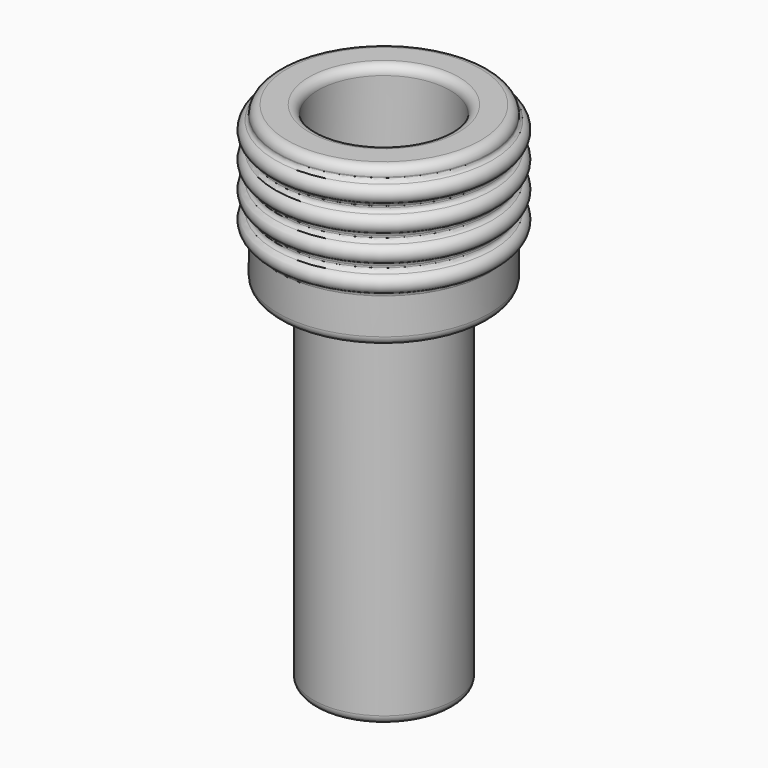
from build123d import *

# Parameters (mm, degrees)
F0_R          = 6
F0_R_2        = 2.05
F1_DEPTH      = 4
F2_R          = 6
F2_R_2        = 3.75
F3_DEPTH      = 5
F4_R          = 0.5
F5_R          = 4
F5_R_2        = 2.05
F6_DEPTH      = 20
F7_R          = 0.5
F10_T3_ANGLE  = 180
F10_T6_ANGLE  = 180
F10_T9_ANGLE  = 180
F10_T12_ANGLE = 180
F10_T15_ANGLE = 180
F10_T18_ANGLE = 180
F10_T21_ANGLE = 180
F10_T24_ANGLE = 180
F10_T27_ANGLE = 180
F10_T30_ANGLE = 180
F10_T33_ANGLE = 180
F10_T36_ANGLE = 180
F10_T39_ANGLE = 180
F10_T42_ANGLE = 180
F10_T45_ANGLE = 180
F10_T48_ANGLE = 180


# Not quite as in the source:
# - a fillet or chamfer that OpenCascade refuses, or shapes differently, is made with other operations: its cross-section is extruded or revolved along the edge and cut away or added


with BuildPart() as f1:
    # F0 (on Top) → F1 (new body)
    with BuildSketch(Plane.XY):
        Circle(F0_R)
        Circle(F0_R_2, mode=Mode.SUBTRACT)
    extrude(amount=F1_DEPTH)

    # F2 (on face) → F3 (join)
    with BuildSketch(Plane.XY.offset(4)):
        Circle(F2_R)
        Circle(F2_R_2, mode=Mode.SUBTRACT)
    extrude(amount=F3_DEPTH)

    # F4
    f4_edges = [f1.edges().sort_by_distance(p)[0] for p in [
        (-3.75, 0, 4),
        (-2.05, 0, 4),
        (-6, 0, 9),
        (-3.75, 0, 9),
    ]]
    fillet(f4_edges, radius=F4_R)

    # F5 (on face) → F6 (join)
    with BuildSketch(Plane(origin=(0, 0, 0), x_dir=(1, 0, 0), z_dir=(0, 0, -1))):
        Circle(F5_R)
        Circle(F5_R_2, mode=Mode.SUBTRACT)
    extrude(amount=F6_DEPTH)

    # F7
    f7_edges = [f1.edges().sort_by_distance(p)[0] for p in [
        (-6, 0, 0),
        (-4, 0, 0),
        (-4, 0, -20),
        (-2.05, 0, -20),
    ]]
    fillet(f7_edges, radius=F7_R)

    # F8 (on Front) → F9 (revolve)
    with BuildSketch(Plane.XZ):
        with BuildLine():
            ThreePointArc((-6, 3.75), (-6.5, 3.25), (-6, 2.75))
            Line((-6, 2.75), (-6, 3.75))
        make_face()
        with BuildLine():
            ThreePointArc((-6, 8.25), (-6.5, 7.75), (-6, 7.25))
            Line((-6, 7.25), (-6, 8.25))
        make_face()
        with BuildLine():
            Line((-6, 8.25), (-6, 7.25))
            ThreePointArc((-6, 7.25), (-5.6464466094, 7.3964466094), (-5.5, 7.75))
            ThreePointArc((-5.5, 7.75), (-5.6464466094, 8.1035533906), (-6, 8.25))
        make_face()
        with BuildLine():
            ThreePointArc((-6, 6.75), (-6.5, 6.25), (-6, 5.75))
            Line((-6, 5.75), (-6, 6.75))
        make_face()
        with BuildLine():
            Line((-6, 6.75), (-6, 5.75))
            ThreePointArc((-6, 5.75), (-5.6464466094, 5.8964466094), (-5.5, 6.25))
            ThreePointArc((-5.5, 6.25), (-5.6464466094, 6.6035533906), (-6, 6.75))
        make_face()
        with BuildLine():
            ThreePointArc((-6, 5.25), (-6.5, 4.75), (-6, 4.25))
            Line((-6, 4.25), (-6, 5.25))
        make_face()
        with BuildLine():
            Line((-6, 5.25), (-6, 4.25))
            ThreePointArc((-6, 4.25), (-5.6464466094, 4.3964466094), (-5.5, 4.75))
            ThreePointArc((-5.5, 4.75), (-5.6464466094, 5.1035533906), (-6, 5.25))
        make_face()
        with BuildLine():
            Line((-6, 3.75), (-6, 2.75))
            ThreePointArc((-6, 2.75), (-5.6464466094, 2.8964466094), (-5.5, 3.25))
            ThreePointArc((-5.5, 3.25), (-5.6464466094, 3.6035533906), (-6, 3.75))
        make_face()
    revolve(axis=Axis((0, 0, 0), (0, 0, -1)))

    # F10: fillet of radius 0.25 on 23 edges, made by hand


with BuildPart() as f10_tool1:
    # F10_s2 → F10_t3 (revolve)
    with BuildSketch(Plane.XZ):
        with BuildLine():
            ThreePointArc((-6.1666666667, 6.7214045208), (-6.0458758548, 6.8127692139), (-6, 6.9571067812))
            Line((-6, 6.9571067812), (-6, 6.75))
            ThreePointArc((-6, 6.75), (-6.0845509894, 6.7427992798), (-6.1666666667, 6.7214045208))
        make_face()
    revolve(axis=Axis((0, 0, 6.75), (0, 0, -1)), revolution_arc=F10_T3_ANGLE)


with BuildPart() as f10_tool4:
    # F10_s5 → F10_t6 (revolve)
    with BuildSketch(Plane.XZ):
        with BuildLine():
            ThreePointArc((6.1666666667, 6.7214045208), (6.0458758548, 6.8127692139), (6, 6.9571067812))
            Line((6, 6.9571067812), (6, 6.75))
            ThreePointArc((6, 6.75), (6.0845509894, 6.7427992798), (6.1666666667, 6.7214045208))
        make_face()
    revolve(axis=Axis((0, 0, 6.75), (0, 0, -1)), revolution_arc=F10_T6_ANGLE)


with BuildPart() as f10_tool7:
    # F10_s8 → F10_t9 (revolve)
    with BuildSketch(Plane.XZ):
        with BuildLine():
            ThreePointArc((6, 7.0428932188), (6.0458758548, 7.1872307861), (6.1666666667, 7.2785954792))
            ThreePointArc((6.1666666667, 7.2785954792), (6.0845509894, 7.2572007202), (6, 7.25))
            Line((6, 7.25), (6, 7.0428932188))
        make_face()
    revolve(axis=Axis((0, 0, 7.25), (0, 0, -1)), revolution_arc=F10_T9_ANGLE)


with BuildPart() as f10_tool10:
    # F10_s11 → F10_t12 (revolve)
    with BuildSketch(Plane.XZ):
        with BuildLine():
            ThreePointArc((-6, 7.0428932188), (-6.0458758548, 7.1872307861), (-6.1666666667, 7.2785954792))
            ThreePointArc((-6.1666666667, 7.2785954792), (-6.0845509894, 7.2572007202), (-6, 7.25))
            Line((-6, 7.25), (-6, 7.0428932188))
        make_face()
    revolve(axis=Axis((0, 0, 7.25), (0, 0, -1)), revolution_arc=F10_T12_ANGLE)


with BuildPart() as f10_tool13:
    # F10_s14 → F10_t15 (revolve)
    with BuildSketch(Plane.XZ):
        with BuildLine():
            ThreePointArc((-6.1666666667, 5.2214045208), (-6.0458758548, 5.3127692139), (-6, 5.4571067812))
            Line((-6, 5.4571067812), (-6, 5.25))
            ThreePointArc((-6, 5.25), (-6.0845509894, 5.2427992798), (-6.1666666667, 5.2214045208))
        make_face()
    revolve(axis=Axis((0, 0, 5.25), (0, 0, -1)), revolution_arc=F10_T15_ANGLE)


with BuildPart() as f10_tool16:
    # F10_s17 → F10_t18 (revolve)
    with BuildSketch(Plane.XZ):
        with BuildLine():
            ThreePointArc((6.1666666667, 5.2214045208), (6.0458758548, 5.3127692139), (6, 5.4571067812))
            Line((6, 5.4571067812), (6, 5.25))
            ThreePointArc((6, 5.25), (6.0845509894, 5.2427992798), (6.1666666667, 5.2214045208))
        make_face()
    revolve(axis=Axis((0, 0, 5.25), (0, 0, -1)), revolution_arc=F10_T18_ANGLE)


with BuildPart() as f10_tool19:
    # F10_s20 → F10_t21 (revolve)
    with BuildSketch(Plane.XZ):
        with BuildLine():
            ThreePointArc((6, 5.5428932188), (6.0458758548, 5.6872307861), (6.1666666667, 5.7785954792))
            ThreePointArc((6.1666666667, 5.7785954792), (6.0845509894, 5.7572007202), (6, 5.75))
            Line((6, 5.75), (6, 5.5428932188))
        make_face()
    revolve(axis=Axis((0, 0, 5.75), (0, 0, -1)), revolution_arc=F10_T21_ANGLE)


with BuildPart() as f10_tool22:
    # F10_s23 → F10_t24 (revolve)
    with BuildSketch(Plane.XZ):
        with BuildLine():
            ThreePointArc((-6, 5.5428932188), (-6.0458758548, 5.6872307861), (-6.1666666667, 5.7785954792))
            ThreePointArc((-6.1666666667, 5.7785954792), (-6.0845509894, 5.7572007202), (-6, 5.75))
            Line((-6, 5.75), (-6, 5.5428932188))
        make_face()
    revolve(axis=Axis((0, 0, 5.75), (0, 0, -1)), revolution_arc=F10_T24_ANGLE)


with BuildPart() as f10_tool25:
    # F10_s26 → F10_t27 (revolve)
    with BuildSketch(Plane.XZ):
        with BuildLine():
            ThreePointArc((-6.1666666667, 3.7214045208), (-6.0458758548, 3.8127692139), (-6, 3.9571067812))
            Line((-6, 3.9571067812), (-6, 3.75))
            ThreePointArc((-6, 3.75), (-6.0845509894, 3.7427992798), (-6.1666666667, 3.7214045208))
        make_face()
    revolve(axis=Axis((0, 0, 3.75), (0, 0, -1)), revolution_arc=F10_T27_ANGLE)


with BuildPart() as f10_tool28:
    # F10_s29 → F10_t30 (revolve)
    with BuildSketch(Plane.XZ):
        with BuildLine():
            ThreePointArc((6.1666666667, 3.7214045208), (6.0458758548, 3.8127692139), (6, 3.9571067812))
            Line((6, 3.9571067812), (6, 3.75))
            ThreePointArc((6, 3.75), (6.0845509894, 3.7427992798), (6.1666666667, 3.7214045208))
        make_face()
    revolve(axis=Axis((0, 0, 3.75), (0, 0, -1)), revolution_arc=F10_T30_ANGLE)


with BuildPart() as f10_tool31:
    # F10_s32 → F10_t33 (revolve)
    with BuildSketch(Plane.XZ):
        with BuildLine():
            ThreePointArc((6, 4.0428932188), (6.0458758548, 4.1872307861), (6.1666666667, 4.2785954792))
            ThreePointArc((6.1666666667, 4.2785954792), (6.0845509894, 4.2572007202), (6, 4.25))
            Line((6, 4.25), (6, 4.0428932188))
        make_face()
    revolve(axis=Axis((0, 0, 4.25), (0, 0, -1)), revolution_arc=F10_T33_ANGLE)


with BuildPart() as f10_tool34:
    # F10_s35 → F10_t36 (revolve)
    with BuildSketch(Plane.XZ):
        with BuildLine():
            ThreePointArc((-6, 4.0428932188), (-6.0458758548, 4.1872307861), (-6.1666666667, 4.2785954792))
            ThreePointArc((-6.1666666667, 4.2785954792), (-6.0845509894, 4.2572007202), (-6, 4.25))
            Line((-6, 4.25), (-6, 4.0428932188))
        make_face()
    revolve(axis=Axis((0, 0, 4.25), (0, 0, -1)), revolution_arc=F10_T36_ANGLE)


with BuildPart() as f10_tool37:
    # F10_s38 → F10_t39 (revolve)
    with BuildSketch(Plane.XZ):
        with BuildLine():
            ThreePointArc((6, 2.5428932188), (6.0458758548, 2.6872307861), (6.1666666667, 2.7785954792))
            ThreePointArc((6.1666666667, 2.7785954792), (6.0845509894, 2.7572007202), (6, 2.75))
            Line((6, 2.75), (6, 2.5428932188))
        make_face()
    revolve(axis=Axis((0, 0, 2.75), (0, 0, -1)), revolution_arc=F10_T39_ANGLE)


with BuildPart() as f10_tool40:
    # F10_s41 → F10_t42 (revolve)
    with BuildSketch(Plane.XZ):
        with BuildLine():
            ThreePointArc((-6, 2.5428932188), (-6.0458758548, 2.6872307861), (-6.1666666667, 2.7785954792))
            ThreePointArc((-6.1666666667, 2.7785954792), (-6.0845509894, 2.7572007202), (-6, 2.75))
            Line((-6, 2.75), (-6, 2.5428932188))
        make_face()
    revolve(axis=Axis((0, 0, 2.75), (0, 0, -1)), revolution_arc=F10_T42_ANGLE)


with BuildPart() as f10_tool43:
    # F10_s44 → F10_t45 (revolve)
    with BuildSketch(Plane.XZ):
        with BuildLine():
            ThreePointArc((-6.1666666667, 8.2214045208), (-6.0458758548, 8.3127692139), (-6, 8.4571067812))
            Line((-6, 8.4571067812), (-6, 8.25))
            ThreePointArc((-6, 8.25), (-6.0845509894, 8.2427992798), (-6.1666666667, 8.2214045208))
        make_face()
    revolve(axis=Axis((0, 0, 8.25), (0, 0, -1)), revolution_arc=F10_T45_ANGLE)


with BuildPart() as f10_tool46:
    # F10_s47 → F10_t48 (revolve)
    with BuildSketch(Plane.XZ):
        with BuildLine():
            ThreePointArc((6.1666666667, 8.2214045208), (6.0458758548, 8.3127692139), (6, 8.4571067812))
            Line((6, 8.4571067812), (6, 8.25))
            ThreePointArc((6, 8.25), (6.0845509894, 8.2427992798), (6.1666666667, 8.2214045208))
        make_face()
    revolve(axis=Axis((0, 0, 8.25), (0, 0, -1)), revolution_arc=F10_T48_ANGLE)


with BuildPart() as f1_1:
    add(f1.part)

    # F10_t49: union F10_tool1, F10_tool4, F10_tool7, F10_tool10, F10_tool13, F10_tool16, F10_tool19, F10_tool22, F10_tool25, F10_tool28, F10_tool31, F10_tool34, F10_tool37, F10_tool40, F10_tool43, F10_tool46
    add([f10_tool1.part, f10_tool4.part, f10_tool7.part, f10_tool10.part, f10_tool13.part, f10_tool16.part, f10_tool19.part, f10_tool22.part, f10_tool25.part, f10_tool28.part, f10_tool31.part, f10_tool34.part, f10_tool37.part, f10_tool40.part, f10_tool43.part, f10_tool46.part])


solid = f1_1.part
